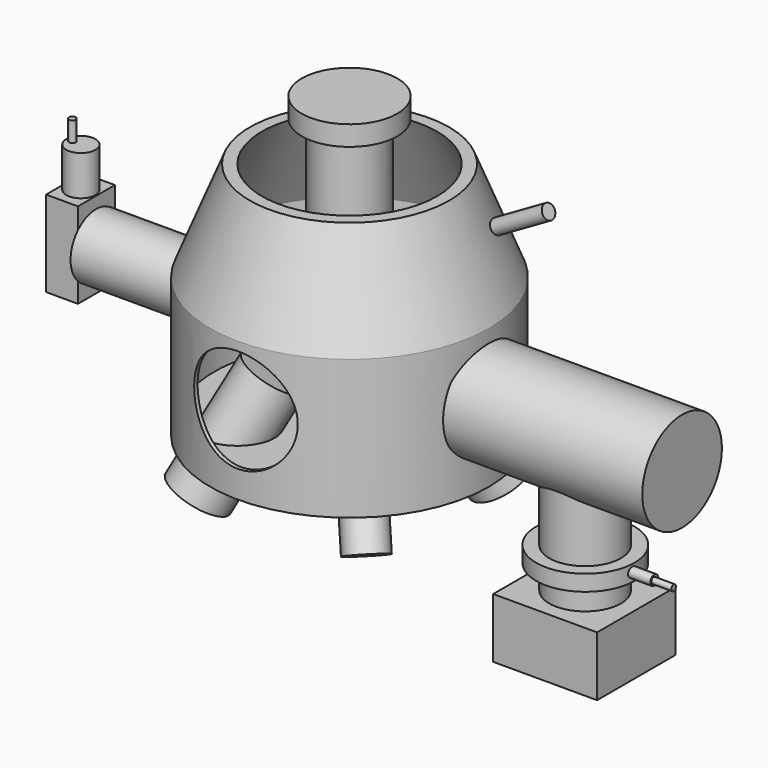
from build123d import *

# Parameters (mm, degrees)
F0_R       = 88.9
F1_DEPTH   = 88.9
F2_R       = 86.36
F3_DEPTH   = 81.28
F7_R       = 12.7
F8_DEPTH   = 76.2
F10_R      = 19.05
F11_DEPTH  = 76.2
F13_R      = 12.7
F14_DEPTH  = 76.2
F16_R      = 19.05
F17_DEPTH  = 76.2
F19_R      = 21.59
F20_DEPTH  = 114.3
F21_R      = 30.48
F22_DEPTH  = 12.7
F24_R      = 63.5
F25_R      = 55.88
F27_FACE_R = 21.59
F30_R      = 20.32
F31_DEPTH  = 76.2
F33_R      = 31.75
F34_DEPTH  = 127
F35_R      = 22.86
F36_DEPTH  = 76.2
F38_R      = 33.02
F39_DEPTH  = 12.7
F41_R      = 3.556
F43_DEPTH  = 12.7
F42_R      = 3.556
F44_DEPTH  = 12.7
F47_R      = 31.3505645065
F48_DEPTH  = 10.16
F50_R      = 3.173998601
F51_DEPTH  = 17.78
F52_R      = 1.905
F53_DEPTH  = 30.48
F55_R      = 29.310353423
F56_DEPTH  = 2.54
F58_R      = 18.968209012
F59_DEPTH  = 2.032
F61_W      = 66.2369132042
F61_H      = 62.4734573066
F62_DEPTH  = 38.1
F64_W      = 29.4773610658
F64_H      = 54.7436773777
F65_DEPTH  = 20.32
F67_R      = 9.2871625742
F68_DEPTH  = 25.4
F69_R      = 2.1469420822
F70_DEPTH  = 12.7
F73_R      = 4.6003508231
F74_DEPTH  = 38.1


with BuildPart() as f1:
    # F0 (on Top) → F1 (new body)
    with BuildSketch(Plane.XY):
        Circle(F0_R)
    extrude(amount=-F1_DEPTH)

    # F2 (on face) → F3 (cut)
    with BuildSketch(Plane.XY):
        Circle(F2_R)
    extrude(amount=-F3_DEPTH, mode=Mode.SUBTRACT)

    # F7 (on face) → F8 (join)
    with BuildSketch(Plane(origin=(-22.2894519575, 22.2894519575, -54.5977839421), x_dir=(0.9354143467, 0.133630621, -0.3273268354), z_dir=(0.3535533906, -0.3535533906, 0.8660254038))):
        with Locations((-5.4411096498, 5.5057285354)):
            Circle(F7_R)
    extrude(amount=-F8_DEPTH)

    # F10 (on face) → F11 (join)
    with BuildSketch(Plane(origin=(-22.2894519575, -22.2894519575, -54.5977839421), x_dir=(0.9354143467, -0.133630621, -0.3273268354), z_dir=(0.3535533906, 0.3535533906, 0.8660254038))):
        with Locations((-4.3192654848, -6.0806246474)):
            Circle(F10_R)
    extrude(amount=-F11_DEPTH)

    # F13 (on face) → F14 (join)
    with BuildSketch(Plane(origin=(22.2894519575, -22.2894519575, -54.5977839421), x_dir=(0.9354143467, 0.133630621, 0.3273268354), z_dir=(0.3535533906, -0.3535533906, -0.8660254038))):
        with Locations((4.7596194781, 5.515140947)):
            Circle(F13_R)
    extrude(amount=F14_DEPTH)

    # F16 (on face) → F17 (join)
    with BuildSketch(Plane(origin=(22.2894519575, 22.2894519575, -54.5977839421), x_dir=(0.9354143467, -0.133630621, 0.3273268354), z_dir=(0.3535533906, 0.3535533906, -0.8660254038))):
        with Locations((4.6711470932, -5.7632611133)):
            Circle(F16_R)
    extrude(amount=F17_DEPTH)

    # F33 (on offset) → F34 (join)
    with BuildSketch(Plane.YZ.offset(85.09)):
        with Locations((0, -40.0666470004)):
            Circle(F33_R)
    extrude(amount=F34_DEPTH)

    # F35 (on offset) → F36 (join)
    with BuildSketch(Plane.XY.offset(-50.8)):
        with Locations((150.2468418311, 0)):
            Circle(F35_R)
    extrude(amount=-F36_DEPTH)

    # F38 (on offset) → F39 (cut)
    with BuildSketch(Plane.XZ.offset(88.9)):
        with Locations((0, -38.5895837275)):
            Circle(F38_R)
    extrude(amount=-F39_DEPTH, mode=Mode.SUBTRACT)

    # F47 (on offset) → F48 (join)
    with BuildSketch(Plane(origin=(0, 0, -101.6), x_dir=(1, 0, 0), z_dir=(0, 0, -1))):
        with Locations((150.114223361, -0.3355145745)):
            Circle(F47_R)
    extrude(amount=F48_DEPTH)

    # F50 (on offset) → F51 (join)
    with BuildSketch(Plane.YZ.offset(177.546)):
        with Locations((-1.1955500813, -106.1796322465)):
            Circle(F50_R)
    extrude(amount=F51_DEPTH)

    # F52 (on offset) → F53 (join)
    with BuildSketch(Plane.YZ.offset(177.546)):
        with Locations((-1.6459240578, -106.1796322465)):
            Circle(F52_R)
    extrude(amount=F53_DEPTH)

    # F61 (on offset) → F62 (join)
    with BuildSketch(Plane(origin=(0, 0, -165.1), x_dir=(1, 0, 0), z_dir=(0, 0, -1))):
        with Locations((150.1587480307, 0.5213841796)):
            Rectangle(F61_W, F61_H)
    extrude(amount=-F62_DEPTH)


with BuildPart() as f20:
    # F19 (on offset) → F20 (new body)
    with BuildSketch(Plane.XY.offset(88.9)):
        Circle(F19_R)
    extrude(amount=-F20_DEPTH)

    # F21 (on offset) → F22 (join)
    with BuildSketch(Plane.XY.offset(88.9)):
        Circle(F21_R)
    extrude(amount=F22_DEPTH)


with BuildPart() as f26:
    # F24 (on offset) → F26 section 0
    with BuildSketch(Plane.XY.offset(63.5)):
        Circle(F24_R)
    # F0 (on Top) → F26 section 1
    with BuildSketch(Plane.XY):
        Circle(F0_R)
    loft()


with BuildPart() as f27_tool:
    # F25 (on offset) → F27 section 0
    with BuildSketch(Plane.XY.offset(63.5)):
        Circle(F25_R)
    # F2 (on face) → F27 section 1
    with BuildSketch(Plane.XY):
        Circle(F2_R)
    loft()


with BuildPart() as f20_1:
    add(f20.part)

    # F27: cut by f27_tool
    add(f27_tool.part, mode=Mode.SUBTRACT)


with BuildPart() as f26_1:
    add(f26.part)

    # F27: cut by f27_tool
    add(f27_tool.part, mode=Mode.SUBTRACT)


with BuildPart() as f28:
    # F19 (on offset) → F28 section 0
    with BuildSketch(Plane.XY.offset(88.9)):
        Circle(F19_R)
    # F27_face (on face) → F28 section 1
    with BuildSketch(Plane.XY):
        Circle(F27_FACE_R)
    loft()


with BuildPart() as f31:
    # F30 (on offset) → F31 (new body)
    with BuildSketch(Plane.YZ.offset(-85.09)):
        with Locations((-0.4500148934, -34.4532616436)):
            Circle(F30_R)
    extrude(amount=-F31_DEPTH)

    # F64 (on offset) → F65 (join)
    with BuildSketch(Plane(origin=(-181.61, 0, 0), x_dir=(0, -1, 0), z_dir=(-1, 0, 0))):
        with Locations((0.138754287, -34.1187156737)):
            Rectangle(F64_W, F64_H)
    extrude(amount=-F65_DEPTH)


with BuildPart() as f43:
    # F41 (on offset) → F43 (new body)
    with BuildSketch(Plane.XZ.offset(-88.646)):
        with Locations((20.4399116337, -39.2765179276)):
            Circle(F41_R)
    extrude(amount=-F43_DEPTH)


with BuildPart() as f44:
    # F42 (on offset) → F44 (new body)
    with BuildSketch(Plane.XZ.offset(-88.646)):
        with Locations((-16.6505910456, -38.8349629939)):
            Circle(F42_R)
    extrude(amount=-F44_DEPTH)


with BuildPart() as f56:
    # F55 (on offset) → F56 (new body)
    with BuildSketch(Plane.XY.offset(-33.528)):
        with Locations((-0.2945478482, 0.2245975047)):
            Circle(F55_R)
    extrude(amount=F56_DEPTH)


with BuildPart() as f59:
    # F58 (on offset) → F59 (new body)
    with BuildSketch(Plane(origin=(19.5953751212, 19.5953751212, -47.9986703653), x_dir=(0.9354143467, -0.133630621, 0.3273268354), z_dir=(0.3535533906, 0.3535533906, -0.8660254038))):
        with Locations((3.652572399, -4.896286875)):
            Circle(F58_R)
    extrude(amount=-F59_DEPTH)


with BuildPart() as f68:
    # F67 (on offset) → F68 (new body)
    with BuildSketch(Plane.XY.offset(18.6531230152)):
        with Locations((-171.3605970144, 0.0573388606)):
            Circle(F67_R)
    extrude(amount=-F68_DEPTH)

    # F69 (on face) → F70 (join)
    with BuildSketch(Plane.XY.offset(18.6531230152)):
        with Locations((-176.9437640905, 0.2442759869)):
            Circle(F69_R)
    extrude(amount=F70_DEPTH)


with BuildPart() as f74:
    # F73 (on face) → F74 (new body)
    with BuildSketch(Plane(origin=(69.8429465006, 0, 40.3238439631), x_dir=(0, -1, 0), z_dir=(-0.8660254038, 0, -0.5))):
        with Locations((-29.3815713376, -1.1588388588)):
            Circle(F73_R)
    extrude(amount=-F74_DEPTH)


solid = Compound([f1.part, f20_1.part, f26_1.part, f28.part, f31.part, f43.part, f44.part, f56.part, f59.part, f68.part, f74.part])
